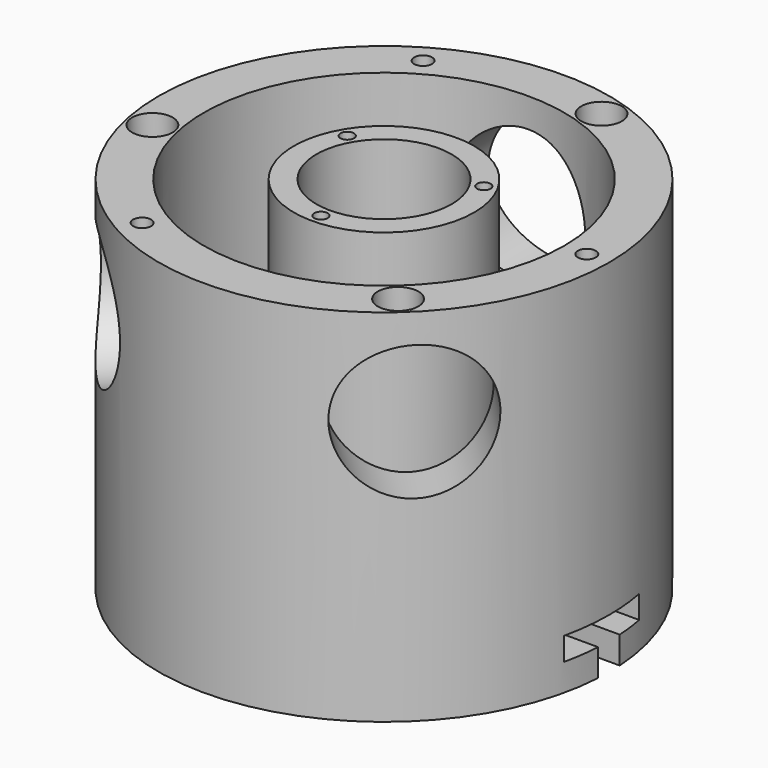
from build123d import *

# Parameters (mm, degrees)
F0_R      = 50
F1_DEPTH  = 40
F2_R      = 40
F3_DEPTH  = 70
F4_R      = 20
F5_DEPTH  = 70
F6_R      = 15
F7_DEPTH  = 70
F8_R      = 4.5
F9_DEPTH  = 5
F10_R     = 3
F11_DEPTH = 3
F12_R     = 3
F13_DEPTH = 5
F14_R     = 3
F15_DEPTH = 5
F16_DEPTH = 5
F17_R     = 2
F18_DEPTH = 25
F19_R     = 1.5
F20_DEPTH = 25
F22_R     = 15
F23_DEPTH = 15
F26_R     = 15
F27_DEPTH = 25
F32_R     = 15
F33_DEPTH = 25
F35_DEPTH = 50
F36_R     = 10.6520252132
F37_DEPTH = 25


with BuildPart() as f1:
    # F0 (on Top) → F1 (new body, symmetric)
    with BuildSketch(Plane.XY):
        Circle(F0_R)
    extrude(amount=F1_DEPTH, both=True)

    # F2 (on face) → F3 (cut)
    with BuildSketch(Plane.XY.offset(40)):
        Circle(F2_R)
    extrude(amount=-F3_DEPTH, mode=Mode.SUBTRACT)

    # F4 (on face) → F5 (join)
    with BuildSketch(Plane.XY.offset(-30)):
        Circle(F4_R)
    extrude(amount=F5_DEPTH)

    # F6 (on face) → F7 (cut)
    with BuildSketch(Plane.XY.offset(40)):
        Circle(F6_R)
    extrude(amount=-F7_DEPTH, mode=Mode.SUBTRACT)

    # F8 (on face) → F9 (cut)
    with BuildSketch(Plane.XY.offset(40)):
        with Locations((-44.0549232574, -9.1740796152)):
            Circle(F8_R)
        with Locations((29.9724476318, -33.5656428951)):
            Circle(F8_R)
        with Locations((14.0824756256, 42.7397225103)):
            Circle(F8_R)
    extrude(amount=-F9_DEPTH, mode=Mode.SUBTRACT)

    # F10 (on face) → F11 (cut)
    with BuildSketch(Plane.XY.offset(35)):
        with Locations((14.0824756256, 42.7397225103)):
            Circle(F10_R)
    extrude(amount=-F11_DEPTH, mode=Mode.SUBTRACT)

    # F12 (on face) → F13 (cut)
    with BuildSketch(Plane.XY.offset(35)):
        with Locations((-44.0549232574, -9.1740796152)):
            Circle(F12_R)
    extrude(amount=-F13_DEPTH, mode=Mode.SUBTRACT)

    # F14 (on face) → F15 (cut)
    with BuildSketch(Plane.XY.offset(35)):
        with Locations((29.9724476318, -33.5656428951)):
            Circle(F14_R)
    extrude(amount=F15_DEPTH, mode=Mode.SUBTRACT)

    # F14 (on face) → F16 (cut)
    with BuildSketch(Plane.XY.offset(35)):
        with Locations((29.9724476318, -33.5656428951)):
            Circle(F14_R)
    extrude(amount=-F16_DEPTH, mode=Mode.SUBTRACT)

    # F17 (on face) → F18 (cut)
    with BuildSketch(Plane.XY.offset(40)):
        with Locations((-22.5, 38.9711431703)):
            Circle(F17_R)
        with Locations((-22.5, -38.9711431703)):
            Circle(F17_R)
        with Locations((45, 0)):
            Circle(F17_R)
    extrude(amount=-F18_DEPTH, mode=Mode.SUBTRACT)

    # F19 (on face) → F20 (cut)
    with BuildSketch(Plane.XY.offset(40)):
        with Locations((-15.1554445662, 8.75)):
            Circle(F19_R)
        with Locations((15.1554445662, 8.75)):
            Circle(F19_R)
        with Locations((0, -17.5)):
            Circle(F19_R)
    extrude(amount=-F20_DEPTH, mode=Mode.SUBTRACT)

    # F22 (on offset) → F23 (cut)
    with BuildSketch(Plane.XZ.offset(-50)):
        with Locations((0, 18.5)):
            Circle(F22_R)
    extrude(amount=F23_DEPTH, mode=Mode.SUBTRACT)

    # F26 (on face) → F27 (cut)
    with BuildSketch(Plane(origin=(-35.3553390593, -35.3553390593, 0), x_dir=(0.7071067812, -0.7071067812, 0), z_dir=(-0.7071067812, -0.7071067812, 0))):
        with Locations((0, 18.5)):
            Circle(F26_R)
    extrude(amount=-F27_DEPTH, mode=Mode.SUBTRACT)

    # F32 (on face) → F33 (cut)
    with BuildSketch(Plane(origin=(35.3553390593, -35.3553390593, 0), x_dir=(0.7071067812, 0.7071067812, 0), z_dir=(0.7071067812, -0.7071067812, 0))):
        with Locations((0, 18.5)):
            Circle(F32_R)
    extrude(amount=-F33_DEPTH, mode=Mode.SUBTRACT)

    # F34 (on offset) → F35 (cut)
    with BuildSketch(Plane.YZ.offset(50)):
        Polygon((-3, -33.9592769742), (-3, -40), (0, -40), (3, -40), (3, -33.9592769742), (9.4083147123, -33.9592769742), (9.4083147123, -28.8467667997), (-10.9889963642, -28.8467667997), (-10.9889963642, -33.9592769742), align=None)
    extrude(amount=-F35_DEPTH, mode=Mode.SUBTRACT)

    # F36 (on face) → F37 (cut)
    with BuildSketch(Plane.XY.offset(-30)):
        Circle(F36_R)
    extrude(amount=-F37_DEPTH, mode=Mode.SUBTRACT)


solid = f1.part
